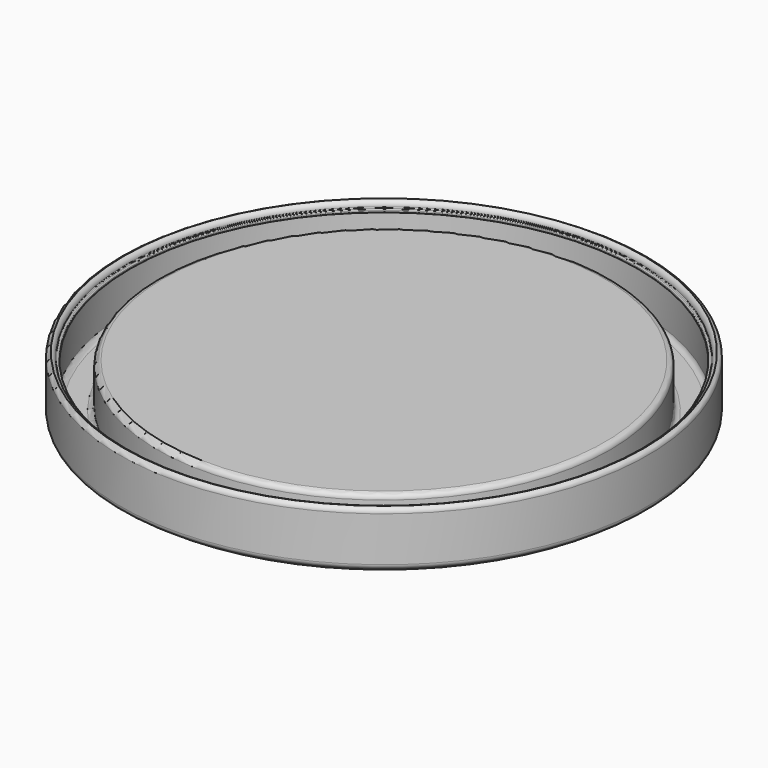
from build123d import *

# Parameters (mm, degrees)
F2_TEXT_SIZE = 19.8757763975
F3_DEPTH     = 2


# Not quite as in the source:
# - Text() gives the source's letters only with a copy of the font that has no kerning and outlines rounded to 1/6400 em; it was checked with that copy


with BuildPart() as f1:
    # F0 (on Front) → F1 (revolve)
    with BuildSketch(Plane.XZ):
        with BuildLine():
            ThreePointArc((-34.4908136561, 7.97342394), (-34.8583839629, 7.7219634897), (-35, 7.2997251842))
            Line((-35, 7.2997251842), (-35, 1.370230158))
            ThreePointArc((-35, 1.370230158), (-34.9188035947, 1.0429279439), (-34.6940437184, 0.7915266836))
            Line((-34.6940437184, 0.7915266836), (-33.7108145509, 0.1215713415))
            ThreePointArc((-33.7108145509, 0.1215713415), (-33.5228129437, 0.0310826586), (-33.3164960167, 0))
            Line((-33.3164960167, 0), (-30, 0))
            Line((-30, 0), (0, 0))
            Line((0, 0), (0, 2.1949816797))
            Line((0, 2.1949816797), (0, 7))
            Line((0, 7), (-29.2997251842, 7))
            ThreePointArc((-29.2997251842, 7), (-29.7948942552, 6.7948942552), (-30, 6.2997251842))
            Line((-30, 6.2997251842), (-30, 1.7002748158))
            ThreePointArc((-30, 1.7002748158), (-30.2051057448, 1.2051057448), (-30.7002748158, 1))
            Line((-30.7002748158, 1), (-33.318097872, 1))
            ThreePointArc((-33.318097872, 1), (-33.7532943153, 1.1516502872), (-34, 1.5409189078))
            Line((-34, 1.5409189078), (-34, 6.6271514663))
            ThreePointArc((-34, 6.6271514663), (-33.9668316346, 6.7072269838), (-33.8867561171, 6.7403953492))
            Line((-33.8867561171, 6.7403953492), (-33.7132438829, 6.7403953492))
            ThreePointArc((-33.7132438829, 6.7403953492), (-33.6331683654, 6.7735637145), (-33.6, 6.853639232))
            Line((-33.6, 6.853639232), (-33.6, 7.0271253934))
            ThreePointArc((-33.6, 7.0271253934), (-33.6331683654, 7.1072009109), (-33.7132438829, 7.1403692762))
            Line((-33.7132438829, 7.1403692762), (-33.8946765933, 7.1403692762))
            ThreePointArc((-33.8946765933, 7.1403692762), (-33.9610500453, 7.1695863438), (-33.9843293277, 7.2382678345))
            ThreePointArc((-33.9843293277, 7.2382678345), (-34.1052364198, 7.6970178705), (-34.4908136561, 7.97342394))
        make_face()
    revolve(axis=Axis((0, 0, 1.0974908398), (0, 0, -1)))

    # F2 (on face) → F3 (cut)
    with BuildSketch(Plane(origin=(0, 0, 0), x_dir=(1, 0, 0), z_dir=(0, 0, -1))):
        with Locations((-25, -6.803585314)):
            Text('2o3A', F2_TEXT_SIZE, font='Open Sans', font_style=FontStyle.BOLD, text_align=(TextAlign.LEFT, TextAlign.BOTTOM))
    extrude(amount=-F3_DEPTH, mode=Mode.SUBTRACT)


solid = f1.part
